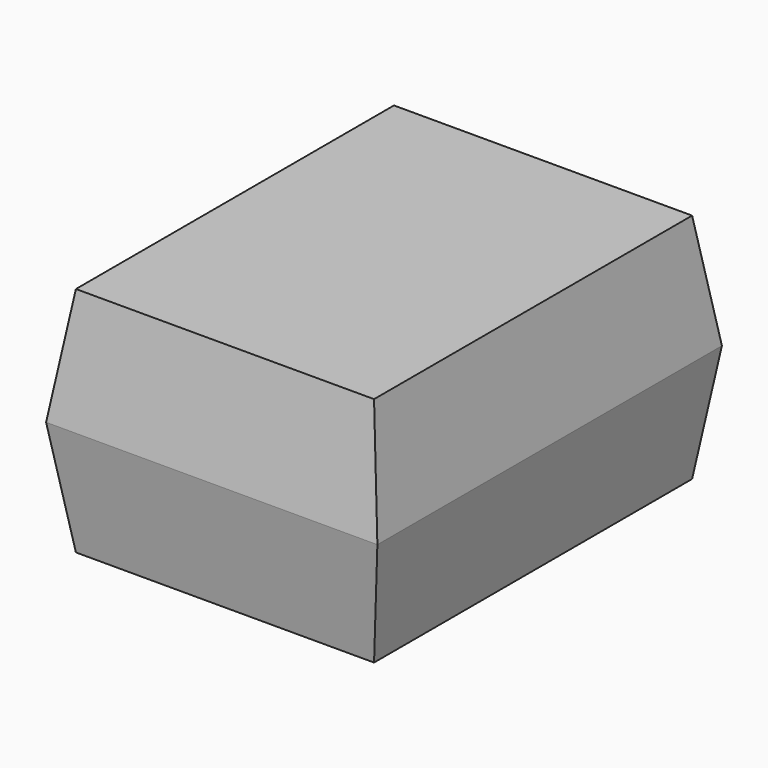
from build123d import *

# Parameters (mm, degrees)
F0_W        = 10
F0_H        = 13
F1_DEPTH    = 7
F2_T1_DEPTH = 31.1932339785
F2_T3_DEPTH = 28.1932339785


# Not quite as in the source:
# - a fillet or chamfer that OpenCascade refuses, or shapes differently, is made with other operations: its cross-section is extruded or revolved along the edge and cut away or added
# - a feature of the source that left no trace in its solid (it failed there, or was rolled back) is left out


with BuildPart() as f1:
    # F0 (on Top) → F1 (new body)
    with BuildSketch(Plane.XY):
        Rectangle(F0_W, F0_H)
    extrude(amount=F1_DEPTH)

    # F2: chamfer of 0.5 x 3.5 on 8 edges, made by hand

    # F2_s2 → F2_t1 (cut)
    with BuildSketch(Plane.XZ.offset(-15.5966169892)):
        Polygon((-5, 3.5), (-4.5, 7), (-5, 7), align=None)
        Polygon((5, 3.5), (4.5, 7), (5, 7), align=None)
        Polygon((-5, 3.5), (-4.5, 0), (-5, 0), align=None)
        Polygon((5, 3.5), (4.5, 0), (5, 0), align=None)
    extrude(amount=F2_T1_DEPTH, mode=Mode.SUBTRACT)

    # F2_s4 → F2_t3 (cut)
    with BuildSketch(Plane.YZ.offset(-14.0966169892)):
        Polygon((-6.5, 3.5), (-6, 7), (-6.5, 7), align=None)
        Polygon((6.5, 3.5), (6, 7), (6.5, 7), align=None)
        Polygon((-6.5, 3.5), (-6, 0), (-6.5, 0), align=None)
        Polygon((6.5, 3.5), (6, 0), (6.5, 0), align=None)
    extrude(amount=F2_T3_DEPTH, mode=Mode.SUBTRACT)


solid = f1.part
